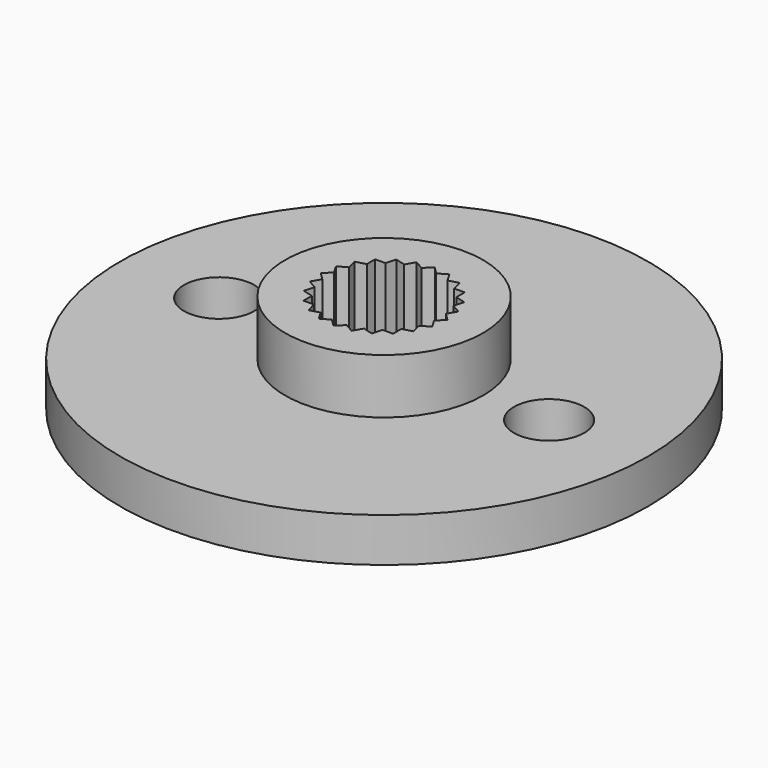
from build123d import *

# Parameters (mm, degrees)
F0_R            = 12
F1_DEPTH        = 2
F2_R            = 4.5
F3_DEPTH        = 2.5
F4_R            = 2.565
F5_DEPTH        = 3
F7_DEPTH        = 3
F7_COPIES_COUNT = 24
F8_R            = 1.25
F9_DEPTH        = 4.501
F10_R           = 1.6
F11_DEPTH       = 2


# Not quite as in the source:
# - a pattern or mirror of a feature is missing from the dataset's text; its kind, count and spacing are read off the source's solid


with BuildPart() as f1:
    # F0 (on Top) → F1 (new body)
    with BuildSketch(Plane.XY):
        Circle(F0_R)
    extrude(amount=F1_DEPTH)

    # F2 (on face) → F3 (join)
    with BuildSketch(Plane.XY.offset(2)):
        Circle(F2_R)
    extrude(amount=F3_DEPTH)

    # F4 (on face) → F5 (cut)
    with BuildSketch(Plane.XY.offset(4.5)):
        Circle(F4_R)
    extrude(amount=-F5_DEPTH, mode=Mode.SUBTRACT)

    # F6 (on face) → F7 (cut, through all)
    with BuildSketch(Plane.XY.offset(4.5)):
        with BuildLine():
            Line((0, 2.88), (-0.334799683, 2.5430560694))
            ThreePointArc((-0.334799683, 2.5430560694), (0, 2.565), (0.334799683, 2.5430560694))
            Line((0.334799683, 2.5430560694), (0, 2.88))
        make_face()
    f7 = extrude(amount=-F7_DEPTH, mode=Mode.SUBTRACT)

    # F7_copies: F7 ×24 about axis
    f7_copies_axis = Axis((0, 0, 0), (0, 0, 1))
    for i in range(1, F7_COPIES_COUNT):
        add(f7.rotate(f7_copies_axis, i * 360 / F7_COPIES_COUNT), mode=Mode.SUBTRACT)

    # F8 (on face) → F9 (cut, through all)
    with BuildSketch(Plane(origin=(0, 0, 0), x_dir=(1, 0, 0), z_dir=(0, 0, -1))):
        Circle(F8_R)
    extrude(amount=-F9_DEPTH, mode=Mode.SUBTRACT)

    # F10 (on face) → F11 (cut, through all)
    with BuildSketch(Plane(origin=(0, 0, 0), x_dir=(1, 0, 0), z_dir=(0, 0, -1))):
        with Locations((-7.5, 0)):
            Circle(F10_R)
        with Locations((7.5, 0)):
            Circle(F10_R)
    extrude(amount=-F11_DEPTH, mode=Mode.SUBTRACT)


solid = f1.part
